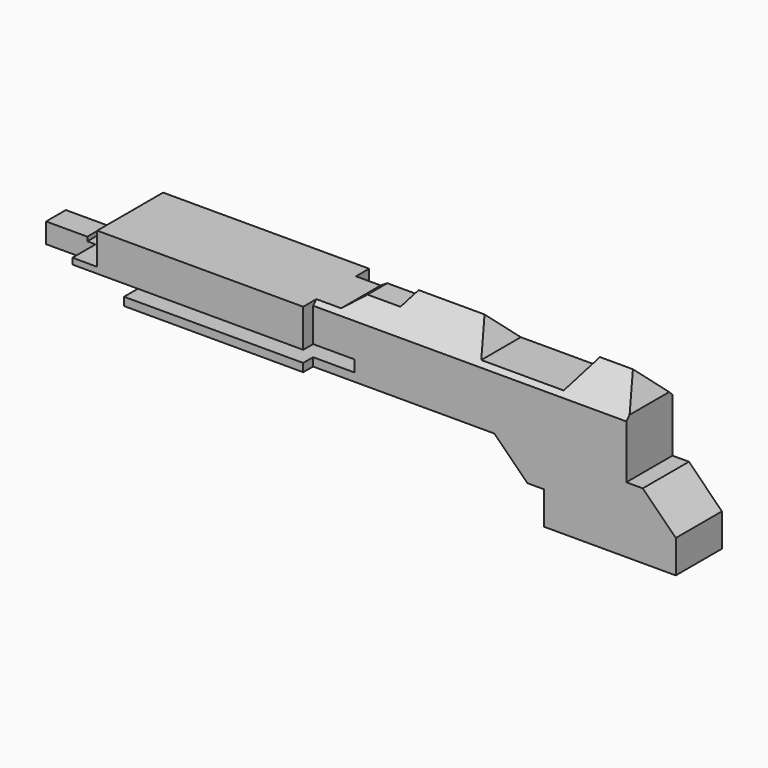
from build123d import *

# Parameters (mm, degrees)
F0_W      = 3
F0_H      = 1.5
F0_W_2    = 2
F0_H_2    = 3.5
F0_W_3    = 1
F0_W_4    = 8
F1_DEPTH  = 9
F5_DEPTH  = 25
F7_DEPTH  = 25
F9_DEPTH  = 25
F10_W     = 3
F10_H     = 0.6
F11_DEPTH = 25
F12_SIZE2 = 1.75
F12_SIZE  = 1.75
F13_SIZE2 = 1.74999
F13_SIZE  = 1.74999


# Not quite as in the source:
# - a fillet or chamfer is up to 0.001 mm smaller than in the source, because OpenCascade refuses the exact size


with BuildPart() as f1:
    # F0 (on Top) → F1 (new body)
    with BuildSketch(Plane.XY):
        Polygon((4.1984589845, 2.5), (-9.8015410155, 2.5), (-9.8015410155, 0.75), (-9.8015410155, -0.75), (-9.8015410155, -2.5), (4.1984589845, -2.5), (4.1984589845, -1.75), (15.1984589845, -1.75), (15.1984589845, 1.75), (4.1984589845, 1.75), align=None)
        with Locations((-11.3015410155, 0)):
            Rectangle(F0_W, F0_H)
        with Locations((16.1984589845, 0)):
            Rectangle(F0_W_2, F0_H_2)
        with Locations((17.6984589845, 0)):
            Rectangle(F0_W_3, F0_H_2)
        with Locations((22.1984589845, 0)):
            Rectangle(F0_W_4, F0_H_2)
    extrude(amount=-F1_DEPTH)

    # F4 (on offset) → F5 (cut)
    with BuildSketch(Plane(origin=(0, 2.5, 0), x_dir=(-1, 0, 0), z_dir=(0, 1, 0))):
        Polygon((-26.1984589845, -7), (-24.1984589845, -5), (-23.1984589845, -5), (-23.1984589845, -1.5), (-22.1984589845, 0), (-26.1984589845, 0), align=None)
        Polygon((-18.1984589845, 0), (-20.1984589845, 0), (-19.1984589845, -1.5), (-18.1984589845, -1.5), align=None)
    extrude(amount=-F5_DEPTH, mode=Mode.SUBTRACT)

    # F6 (on face) → F7 (cut)
    with BuildSketch(Plane.XZ.offset(1.75)):
        Polygon((4.1984589845, -9), (18.1984589845, -9), (18.1984589845, -7), (17.1984589845, -7), (15.1984589845, -5), (4.1984589845, -5), align=None)
        Polygon((8.6984589845, -0.75), (9.1984589845, 0), (4.1984589845, 0), (4.1984589845, -1.5), (5.6984589845, -1.5), (6.6984589845, -0.75), align=None)
        Polygon((15.1984589845, -1.5), (18.1984589845, -1.5), (18.1984589845, 0), (13.1984589845, 0), (14.1984589845, -1.5), align=None)
    extrude(amount=-F7_DEPTH, mode=Mode.SUBTRACT)

    # F8 (on face) → F9 (cut)
    with BuildSketch(Plane.XZ.offset(2.5)):
        Polygon((-12.8015410155, -9), (4.1984589845, -9), (4.1984589845, -5), (-10.3015410155, -5), (-12.8015410155, -5), align=None)
        Polygon((4.1984589845, -1.5), (4.1984589845, 0), (-12.8015410155, 0), (-12.8015410155, -3.1837357674), (-10.3015410155, -3.1837357674), (-10.3015410155, -3.4337357674), (-8.3015410155, -3.4337357674), (-8.3015410155, -1.5), align=None)
    extrude(amount=-F9_DEPTH, mode=Mode.SUBTRACT)

    # F10 (on face) → F11 (cut)
    with BuildSketch(Plane.XZ.offset(2.5)):
        Polygon((-9.8015410155, -5), (-6.6717453301, -5), (-6.6717453301, -4.5), (6.6984589845, -4.5), (6.6984589845, -3.8), (-9.8015410155, -3.8), (-9.8015410155, -4.4), align=None)
        with Locations((-11.3015410155, -4.7)):
            Rectangle(F10_W, F10_H)
    extrude(amount=-F11_DEPTH, mode=Mode.SUBTRACT)

    # F12
    f12_edges = [f1.edges().sort_by_distance(p)[0] for p in [
        (21.198459, -1.75, 0),
    ]]
    chamfer(f12_edges, length=F12_SIZE, length2=F12_SIZE2)

    # F13 (size 1.75 and 1.75 in the source; OpenCascade refuses exactly that, so slightly less here)
    f13_edges = [f1.edges().sort_by_distance(p)[0] for p in [
        (21.198459, 1.75, 0),
    ]]
    chamfer(f13_edges, length=F13_SIZE, length2=F13_SIZE2)


solid = f1.part
